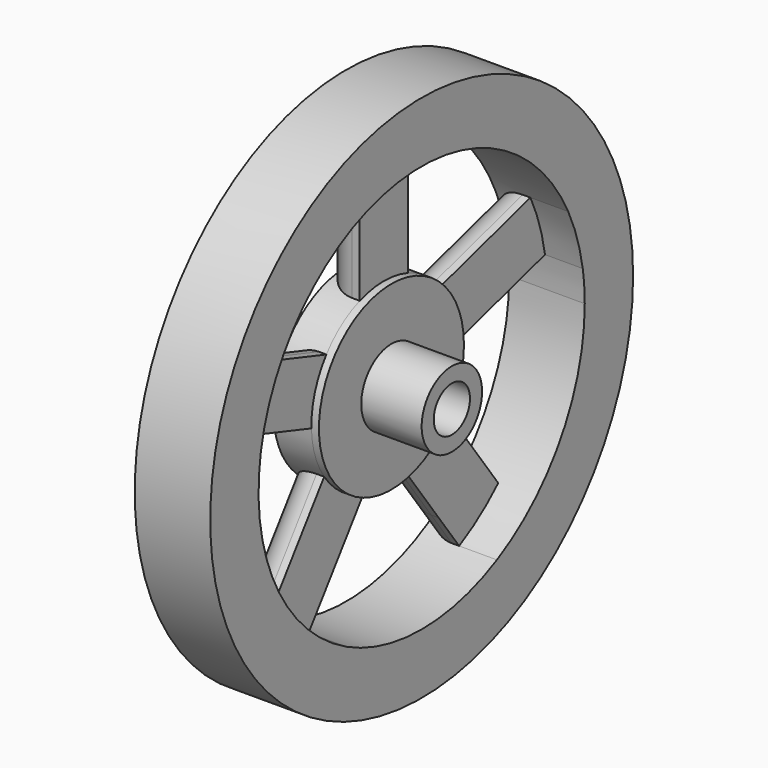
from build123d import *

# Parameters (mm, degrees)
F0_R      = 17.5
F1_DEPTH  = 5
F3_DEPTH  = 25
F4_R      = 13.5
F5_DEPTH  = 2.5
F6_R      = 1.9999
F7_R      = 1.99
F8_R      = 6
F9_DEPTH  = 0.5
F10_R     = 2.5
F11_DEPTH = 4
F12_R     = 1.5
F13_DEPTH = 4.6


# Not quite as in the source:
# - a fillet or chamfer is up to 0.001 mm smaller than in the source, because OpenCascade refuses the exact size


with BuildPart() as f1:
    # F0 (on Right) → F1 (new body)
    with BuildSketch(Plane.YZ):
        Circle(F0_R)
    extrude(amount=F1_DEPTH)

    # F2 (on face) → F3 (cut)
    with BuildSketch(Plane.YZ.offset(5)):
        with BuildLine():
            Line((-2, 5.6568542495), (-2, 13.3510299228))
            ThreePointArc((-2, 13.3510299228), (-7.9351009059, 10.9217294241), (-12.0795500186, 6.0278081711))
            Line((-12.0795500186, 6.0278081711), (-4.761954107, 3.6501771304))
            ThreePointArc((-4.761954107, 3.6501771304), (-3.5267115138, 4.8541019662), (-2, 5.6568542495))
        make_face()
        with BuildLine():
            Line((4.6626960874, 3.7761442234), (12.1273810063, 5.9309889503))
            ThreePointArc((12.1273810063, 5.9309889503), (7.9787201688, 10.8899047042), (2, 13.3510299228))
            Line((2, 13.3510299228), (2, 5.6568542495))
            ThreePointArc((2, 5.6568542495), (3.4615238464, 4.9008012264), (4.6626960874, 3.7761442234))
        make_face()
        with BuildLine():
            ThreePointArc((9.4655724803, -9.6256395954), (12.4506069829, -5.2184658433), (13.5, 0))
            ThreePointArc((13.5, 0), (13.4581864786, 1.0617046234), (13.3330049322, 2.1168324159))
            Line((13.3330049322, 2.1168324159), (6, 0))
            ThreePointArc((6, 0), (5.7296726323, -1.7806884981), (4.943049491, -3.400920718))
            Line((4.943049491, -3.400920718), (7.7712408853, -7.2935922208))
            Line((7.7712408853, -7.2935922208), (9.4655724803, -9.6256395954))
        make_face()
        with BuildLine():
            ThreePointArc((-6.2295045028, -11.9767806046), (0, -13.5), (6.2295045028, -11.9767806046))
            Line((6.2295045028, -11.9767806046), (4.5351729078, -9.64473323))
            Line((4.5351729078, -9.64473323), (1.7069815135, -5.7520617271))
            ThreePointArc((1.7069815135, -5.7520617271), (0, -6), (-1.7069815135, -5.7520617271))
            Line((-1.7069815135, -5.7520617271), (-6.2295045028, -11.9767806046))
        make_face()
        with BuildLine():
            Line((-9.4655724803, -9.6256395954), (-4.943049491, -3.400920718))
            ThreePointArc((-4.943049491, -3.400920718), (-5.7063390978, -1.8541019662), (-5.9980220845, -0.1540489348))
            Line((-5.9980220845, -0.1540489348), (-13.3156179961, 2.223582106))
            ThreePointArc((-13.3156179961, 2.223582106), (-12.83926297, -4.1717294241), (-9.4655724803, -9.6256395954))
        make_face()
    extrude(amount=-F3_DEPTH, mode=Mode.SUBTRACT)

    # F4 (on face) → F5 (cut)
    with BuildSketch(Plane.YZ.offset(5)):
        Circle(F4_R)
    extrude(amount=-F5_DEPTH, mode=Mode.SUBTRACT)

    # F6 (radius 2 in the source; OpenCascade refuses exactly that, so slightly less here)
    f6_edges = [f1.edges().sort_by_distance(p)[0] for p in [
        (0, -9.65682, 1.034767),
        (0, -8.420752, 4.838993),
        (0, -7.204311, -6.51328),
        (0, -3.968243, -8.864421),
        (0, 3.968243, -8.864421),
        (0, 7.204311, -6.51328),
        (0, 9.666502, 1.058416),
        (0, 2, 9.503942),
        (0, -2, 9.503942),
    ]]
    fillet(f6_edges, radius=F6_R)

    # F7
    f7_edges = [f1.edges().sort_by_distance(p)[0] for p in [
        (0, 8.395039, 4.853567),
    ]]
    fillet(f7_edges, radius=F7_R)

    # F8 (on face) → F9 (join)
    with BuildSketch(Plane.YZ.offset(2.5)):
        Circle(F8_R)
    extrude(amount=F9_DEPTH)

    # F10 (on face) → F11 (join)
    with BuildSketch(Plane.YZ.offset(3)):
        Circle(F10_R)
    extrude(amount=F11_DEPTH)

    # F12 (on face) → F13 (cut)
    with BuildSketch(Plane.YZ.offset(7)):
        Circle(F12_R)
    extrude(amount=-F13_DEPTH, mode=Mode.SUBTRACT)


solid = f1.part
